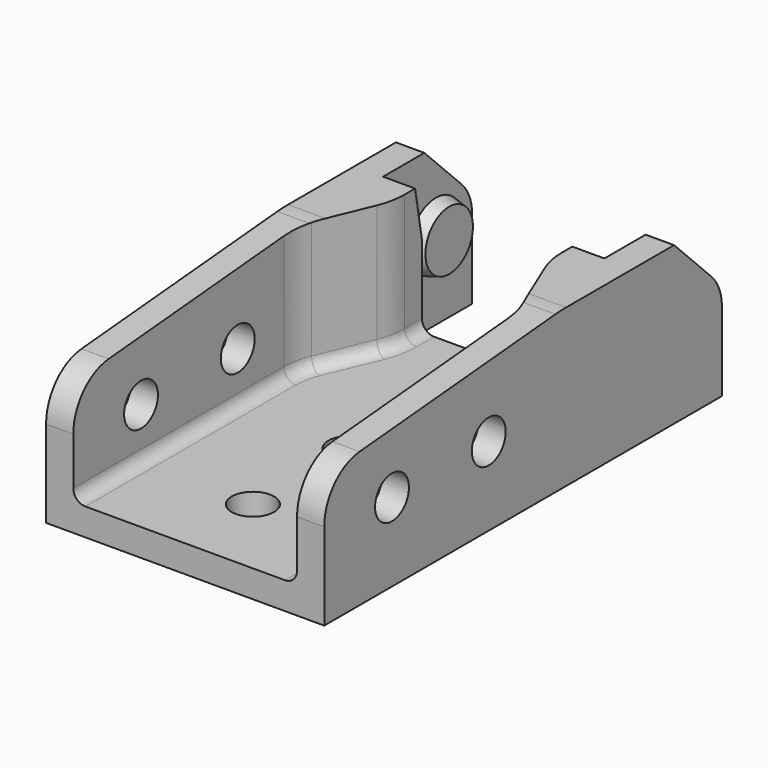
from build123d import *

# Parameters (mm, degrees)
F1_DEPTH      = 13
F2_W          = 13
F2_H          = 10.75
F3_DEPTH      = 38.501
F4_R          = 1.75
F5_DEPTH      = 11.501
F5_DEPTH_BACK = 11.501
F6_R          = 2.75
F7_DEPTH      = 2.65
F8_DEPTH      = 1.55
F8_DEPTH_BACK = 14.55
F9_SIZE2      = 0.294734
F9_SIZE       = 1.09999
F10_DEPTH     = 2.6
F12_DEPTH     = 10.751
F13_R         = 6
F14_R         = 1
F15_R         = 1.75
F16_DEPTH     = 2.251


# Not quite as in the source:
# - a fillet or chamfer is up to 0.001 mm smaller than in the source, because OpenCascade refuses the exact size
# - a pattern or mirror of a feature is missing from the dataset's text; its kind, count and spacing are read off the source's solid


with BuildPart() as f1:
    # F0 (on Top) → F1 (new body)
    with BuildSketch(Plane.XY):
        Polygon((6.5, 30), (0, 30), (-6.5, 30), (-6.5, 38.5), (-11.5, 38.5), (-11.5, -2.6), (-6.5, -2.6), (-6.5, 0), (0, 0), (6.5, 0), (6.5, -2.6), (11.5, -2.6), (11.5, 38.5), (6.5, 38.5), align=None)
    extrude(amount=F1_DEPTH)

    # F2 (on Front) → F3 (cut, through all)
    with BuildSketch(Plane.XZ):
        with Locations((0, 7.625)):
            Rectangle(F2_W, F2_H)
    extrude(amount=-F3_DEPTH, mode=Mode.SUBTRACT)

    # F4 (on Right) → F5 (cut, two sides)
    with BuildSketch(Plane.YZ) as f5_sk:
        with BuildLine():
            Line((38.5, 6.5), (38.5, 13))
            Line((38.5, 13), (33.5533008589, 13))
            Line((33.5533008589, 13), (37.4016504294, 9.1516504294))
            ThreePointArc((37.4016504294, 9.1516504294), (38.2145482469, 7.9350628714), (38.5, 6.5))
        make_face()
        with Locations((4.4, 6.5)):
            Circle(F4_R)
        with Locations((14.4, 6.5)):
            Circle(F4_R)
        with BuildLine():
            ThreePointArc((21.2931220671, 12.9516726658), (21.8460337805, 12.9879124141), (22.4, 13))
            Line((22.4, 13), (-2.6, 13))
            Line((-2.6, 13), (-2.6, 7.1959706526))
            ThreePointArc((-2.6, 7.1959706526), (-1.5491093472, 9.898331483), (1.051377029, 11.1807494449))
            Line((1.051377029, 11.1807494449), (21.2931220671, 12.9516726658))
        make_face()
    extrude(amount=-F5_DEPTH, mode=Mode.SUBTRACT)
    extrude(f5_sk.sketch, amount=F5_DEPTH_BACK, mode=Mode.SUBTRACT)

    # F6 (on face) → F7 (cut)
    with BuildSketch(Plane(origin=(6.5, 0, 0), x_dir=(0, -1, 0), z_dir=(-1, 0, 0))):
        with BuildLine():
            Line((-38.5, 0), (-30, 0))
            Line((-30, 0), (-30, 8.9638140898))
            Line((-30, 8.9638140898), (-29.2883115249, 13))
            Line((-29.2883115249, 13), (-33.5533008589, 13))
            Line((-33.5533008589, 13), (-37.4016504294, 9.1516504294))
            ThreePointArc((-37.4016504294, 9.1516504294), (-38.2145482469, 7.9350628714), (-38.5, 6.5))
            Line((-38.5, 6.5), (-38.5, 0))
        make_face()
        with Locations((-34.75, 6.5)):
            Circle(F6_R, mode=Mode.SUBTRACT)
    f7 = extrude(amount=-F7_DEPTH, mode=Mode.SUBTRACT)

    # F7_copies: F7 across plane
    add(f7.mirror(Plane(origin=(0, 0, 0), x_dir=(0, 0, -1), z_dir=(-1, 0, 0))), mode=Mode.SUBTRACT)

    # F8 (cut, two sides): a face of the model
    f8_faces = [f1.faces().sort_by_distance(p)[0] for p in [
        (6.5, 34.75, 6.5),
    ]]
    extrude(f8_faces, amount=-F8_DEPTH, mode=Mode.SUBTRACT)
    extrude(f8_faces, amount=F8_DEPTH_BACK, mode=Mode.SUBTRACT)

    # F9 (size 1.1 and 0.2947441117 in the source; OpenCascade refuses exactly that, so slightly less here)
    f9_edges = [f1.edges().sort_by_distance(p)[0] for p in [
        (8.05, 37.5, 6.5),
        (-8.05, 37.5, 6.5),
    ]]
    chamfer(f9_edges, length=F9_SIZE, length2=F9_SIZE2)

    # F10 (add, through all): a face of the model
    f10_faces = [f1.faces().sort_by_distance(p)[0] for p in [
        (0, 0, 1.125),
    ]]
    extrude(f10_faces, amount=F10_DEPTH)

    # F11 (on face) → F12 (cut, through all)
    with BuildSketch(Plane.XY.offset(2.25)):
        Polygon((-9.25, -2.6), (9.25, -2.6), (9.25, 20.3609127035), (6.5, 27), (-6.5, 27), (-9.25, 20.3609127035), align=None)
    extrude(amount=F12_DEPTH, mode=Mode.SUBTRACT)

    # F13
    f13_edges = [f1.edges().sort_by_distance(p)[0] for p in [
        (6.5, 27, 7.625),
        (9.25, 20.360913, 7.560057),
        (-6.5, 27, 7.625),
        (-9.25, 20.360913, 7.560057),
    ]]
    fillet(f13_edges, radius=F13_R)

    # F14
    f14_edges = [f1.edges().sort_by_distance(p)[0] for p in [
        (9.25, 8.283719, 2.25),
        (-9.25, 8.283719, 2.25),
        (6.5, 29.096737, 2.25),
        (6.615288, 27.022932, 2.25),
        (7.875, 23.680456, 2.25),
        (-6.5, 29.096737, 2.25),
        (9.134712, 20.33798, 2.25),
        (-6.615288, 27.022932, 2.25),
        (-7.875, 23.680456, 2.25),
        (-9.134712, 20.33798, 2.25),
    ]]
    fillet(f14_edges, radius=F14_R)

    # F15 (on face) → F16 (cut, through all)
    with BuildSketch(Plane.XY.offset(2.25)):
        with Locations((0, 4.4)):
            Circle(F15_R)
        with Locations((0, 14.4)):
            Circle(F15_R)
    extrude(amount=-F16_DEPTH, mode=Mode.SUBTRACT)


solid = f1.part
